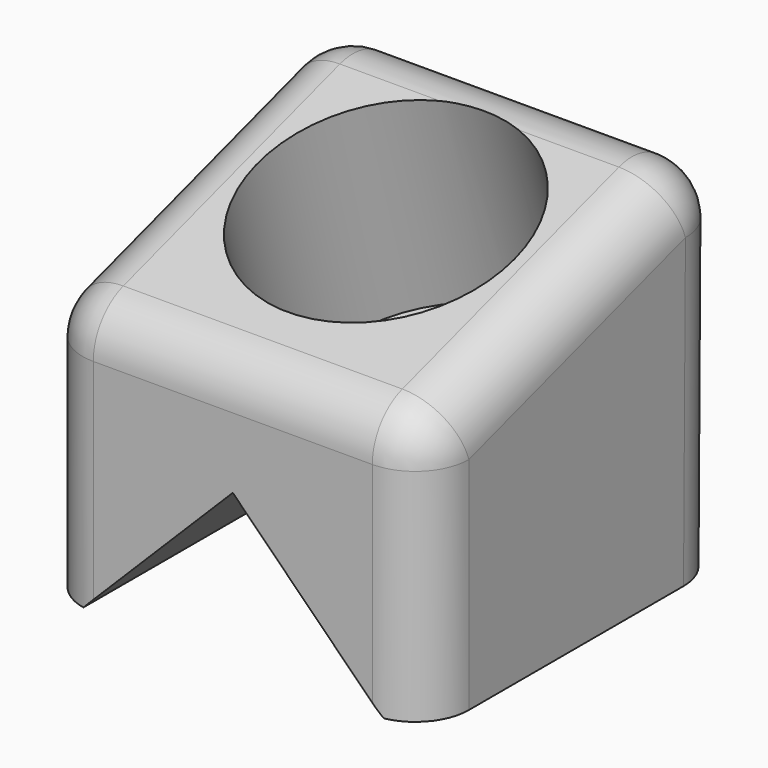
from build123d import *

# Parameters (mm, degrees)
F1_DEPTH     = 18
F2_R         = 12
F3_DEPTH     = 20
F5_DEPTH     = 19
F6_T1_DEPTH  = 33.0501766006
F6_T3_DEPTH  = 26
F6_T5_DEPTH  = 26.4486901769
F6_T7_DEPTH  = 40.9649172436
F6_T12_DEPTH = 5
F6_T18_DEPTH = 5
F6_T24_DEPTH = 5
F6_T30_DEPTH = 5


# Not quite as in the source:
# - a fillet or chamfer that OpenCascade refuses, or shapes differently, is made with other operations: its cross-section is extruded or revolved along the edge and cut away or added


with BuildPart() as f1:
    # F0 (on Right) → F1 (new body, symmetric)
    with BuildSketch(Plane.YZ):
        Polygon((-17.5945106894, -16.5027584881), (17.4054893106, -16.5027584881), (17.6841049034, 18.8368745636), (-17.5945106894, 7.7135697939), align=None)
    extrude(amount=F1_DEPTH, both=True)

    # F2 (on face) → F3 (cut)
    with BuildSketch(Plane(origin=(0, -3.8031265819, 12.0619764999), x_dir=(1, 0, 0), z_dir=(0, -0.3007057995, 0.9537169507))):
        with Locations((0, 4.2350762524)):
            Circle(F2_R)
    extrude(amount=-F3_DEPTH, mode=Mode.SUBTRACT)

    # F4 (on Front) → F5 (cut, symmetric)
    with BuildSketch(Plane.XZ):
        Polygon((18.3847763109, -20.8875347989), (0, -2.5027584881), (-18.3847763109, -20.8875347989), (0, -39.2723111098), align=None)
    extrude(amount=F5_DEPTH, both=True, mode=Mode.SUBTRACT)

    # F6: fillet of radius 5 on 8 edges, made by hand

    # F6_s2 → F6_t1 (cut)
    with BuildSketch(Plane.XY.offset(-29.0027584881)):
        with BuildLine():
            ThreePointArc((-18, -12.5945106894), (-16.5355339059, -16.1300445953), (-13, -17.5945106894))
            Line((-13, -17.5945106894), (-18, -17.5945106894))
            Line((-18, -17.5945106894), (-18, -12.5945106894))
        make_face()
        with BuildLine():
            ThreePointArc((13, -17.5945106894), (16.5355339059, -16.1300445953), (18, -12.5945106894))
            Line((18, -12.5945106894), (18, -17.5945106894))
            Line((18, -17.5945106894), (13, -17.5945106894))
        make_face()
    extrude(amount=F6_T1_DEPTH, mode=Mode.SUBTRACT)

    # F6_s4 → F6_t3 (cut)
    with BuildSketch(Plane.YZ.offset(-13)):
        with BuildLine():
            ThreePointArc((-14.0980396869, 8.8160028663), (-16.6267337107, 7.0039663544), (-17.5945106894, 4.0474181125))
            Line((-17.5945106894, 4.0474181125), (-17.5945106894, 7.7135697939))
            Line((-17.5945106894, 7.7135697939), (-14.0980396869, 8.8160028663))
        make_face()
        with BuildLine():
            ThreePointArc((11.1265244599, 16.7692773918), (15.6024732635, 16.0212299773), (17.6298980733, 11.9612741565))
            Line((17.6298980733, 11.9612741565), (17.6841049034, 18.8368745636))
            Line((17.6841049034, 18.8368745636), (11.1265244599, 16.7692773918))
        make_face()
    extrude(amount=F6_T3_DEPTH, mode=Mode.SUBTRACT)

    # F6_s6 → F6_t5 (cut)
    with BuildSketch(Plane(origin=(0, 14.9296510418, 4.7073008919), x_dir=(1, 0, 0), z_dir=(0, -0.9537169507, -0.3007057995))):
        with BuildLine():
            ThreePointArc((-13, 12.6473336669), (-16.5355339059, 11.1828675728), (-18, 7.6473336669))
            Line((-18, 7.6473336669), (-18, 12.6473336669))
            Line((-18, 12.6473336669), (-13, 12.6473336669))
        make_face()
        with BuildLine():
            ThreePointArc((13, 12.6473336669), (16.5355339059, 11.1828675728), (18, 7.6473336669))
            Line((18, 7.6473336669), (18, 12.6473336669))
            Line((18, 12.6473336669), (13, 12.6473336669))
        make_face()
    extrude(amount=F6_T5_DEPTH, mode=Mode.SUBTRACT)

    # F6_s8 → F6_t7 (cut)
    with BuildSketch(Plane(origin=(0, -0.227563099, -28.8641290101), x_dir=(1, 0, 0), z_dir=(0, 0.0078836963, 0.9999689232))):
        with BuildLine():
            ThreePointArc((13, 17.5350511394), (16.5355339059, 16.0705850454), (18, 12.5350511394))
            Line((18, 12.5350511394), (18, 17.5350511394))
            Line((18, 17.5350511394), (13, 17.5350511394))
        make_face()
        with BuildLine():
            ThreePointArc((-18, 12.5350511394), (-16.5355339059, 16.0705850454), (-13, 17.5350511394))
            Line((-13, 17.5350511394), (-18, 17.5350511394))
            Line((-18, 17.5350511394), (-18, 12.5350511394))
        make_face()
    extrude(amount=F6_T7_DEPTH, mode=Mode.SUBTRACT)


with BuildPart() as f6_tool10:
    # F6_s11 → F6_t12 (new body)
    with BuildSketch(Plane.YZ.offset(-13)):
        Polygon((-12.5945106894, 4.0474181125), (-17.5945106894, 4.0474181125), (-17.5945106894, 7.7135697939), (-14.0980396869, 8.8160028663), align=None)
    extrude(amount=-F6_T12_DEPTH)

    # F6_s13 → F6_t14 (revolve, cut)
    with BuildSketch(Plane(origin=(-13, -12.5945106894, 4.0474181125), x_dir=(0, 0.8064446043, -0.5913096484), z_dir=(0, 0.5913096484, 0.8064446043))):
        with BuildLine():
            ThreePointArc((0, -5), (5, 0), (0, 5))
            Line((0, 5), (0, -5))
        make_face()
    revolve(axis=Axis((-13, -12.5945106894, 4.0474181125), (-1, 0, 0)), mode=Mode.SUBTRACT)


with BuildPart() as f1_1:
    add(f1.part)

    # F6_t9: cut F6_tool10
    add(f6_tool10.part, mode=Mode.SUBTRACT)


with BuildPart() as f6_tool16:
    # F6_s17 → F6_t18 (new body)
    with BuildSketch(Plane.YZ.offset(13)):
        Polygon((-12.5945106894, 4.0474181125), (-14.0980396869, 8.8160028663), (-17.5945106894, 7.7135697939), (-17.5945106894, 4.0474181125), align=None)
    extrude(amount=F6_T18_DEPTH)

    # F6_s19 → F6_t20 (revolve, cut)
    with BuildSketch(Plane(origin=(13, -12.5945106894, 4.0474181125), x_dir=(0, 0.8064446043, -0.5913096484), z_dir=(0, -0.5913096484, -0.8064446043))):
        with BuildLine():
            ThreePointArc((0, -5), (5, 0), (0, 5))
            Line((0, 5), (0, -5))
        make_face()
    revolve(axis=Axis((13, -12.5945106894, 4.0474181125), (1, 0, 0)), mode=Mode.SUBTRACT)


with BuildPart() as f1_2:
    add(f1_1.part)

    # F6_t15: cut F6_tool16
    add(f6_tool16.part, mode=Mode.SUBTRACT)


with BuildPart() as f6_tool22:
    # F6_s23 → F6_t24 (new body)
    with BuildSketch(Plane.YZ.offset(-13)):
        Polygon((12.6300534574, 12.000692638), (17.6298980733, 11.9612741565), (17.6841049034, 18.8368745636), (11.1265244599, 16.7692773918), align=None)
    extrude(amount=-F6_T24_DEPTH)

    # F6_s25 → F6_t26 (revolve, cut)
    with BuildSketch(Plane(origin=(-13, 12.6300534574, 12.000692638), x_dir=(0, -0.5944839612, -0.8041074679), z_dir=(0, 0.8041074679, -0.5944839612))):
        with BuildLine():
            ThreePointArc((0, -5), (5, 0), (0, 5))
            Line((0, 5), (0, -5))
        make_face()
    revolve(axis=Axis((-13, 12.6300534574, 12.000692638), (-1, 0, 0)), mode=Mode.SUBTRACT)


with BuildPart() as f1_3:
    add(f1_2.part)

    # F6_t21: cut F6_tool22
    add(f6_tool22.part, mode=Mode.SUBTRACT)


with BuildPart() as f6_tool28:
    # F6_s29 → F6_t30 (new body)
    with BuildSketch(Plane.YZ.offset(13)):
        Polygon((12.6300534574, 12.000692638), (11.1265244599, 16.7692773918), (17.6841049034, 18.8368745636), (17.6298980733, 11.9612741565), align=None)
    extrude(amount=F6_T30_DEPTH)

    # F6_s31 → F6_t32 (revolve, cut)
    with BuildSketch(Plane(origin=(13, 12.6300534574, 12.000692638), x_dir=(0, -0.5944839612, -0.8041074679), z_dir=(0, -0.8041074679, 0.5944839612))):
        with BuildLine():
            ThreePointArc((0, -5), (5, 0), (0, 5))
            Line((0, 5), (0, -5))
        make_face()
    revolve(axis=Axis((13, 12.6300534574, 12.000692638), (1, 0, 0)), mode=Mode.SUBTRACT)


with BuildPart() as f1_4:
    add(f1_3.part)

    # F6_t27: cut F6_tool28
    add(f6_tool28.part, mode=Mode.SUBTRACT)


solid = f1_4.part
